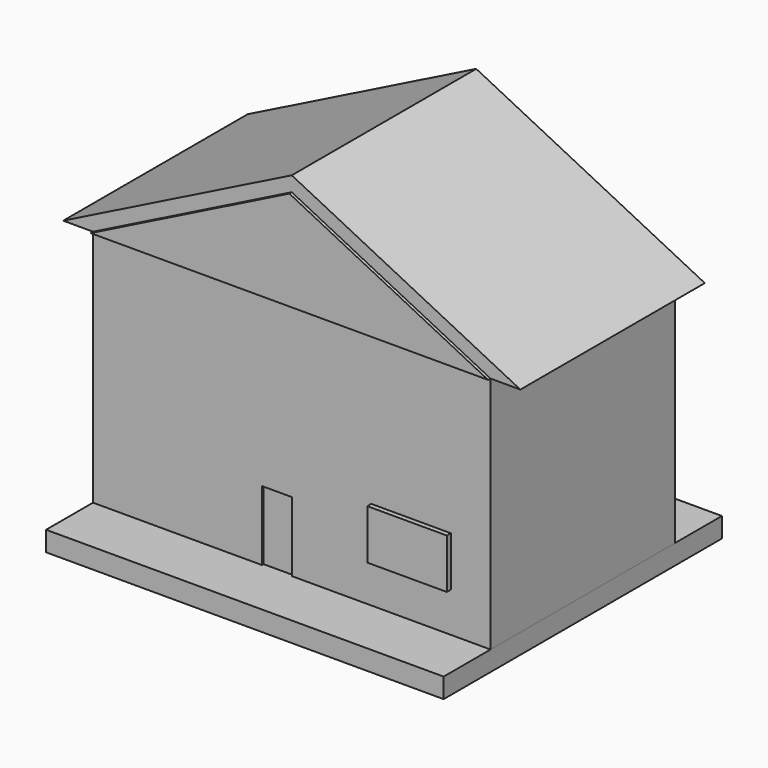
from build123d import *

# Parameters (mm, degrees)
F1_DEPTH     = 1066.8
F2_TEXT_SIZE = 1194.6976415647
F3_DEPTH     = 30.48
F4_DEPTH     = 3535.68
F5_DEPTH     = 3627.12
F0_W         = 2438.4
F0_H         = 1524
F6_DEPTH     = 3535.68
F7_DEPTH     = 5334
F0_W_2       = 914.4
F0_H_2       = 2133.6
F8_DEPTH     = 3474.72
F9_DEPTH     = 3688.08


# Not quite as in the source:
# - Text() gives the source's letters only with a copy of the font that has no kerning and outlines rounded to 1/6400 em; it was checked with that copy


with BuildPart() as f1:
    # F0 (on Front) → F1 (new body)
    with BuildSketch(Plane.XZ):
        Polygon((0, -609.6), (0, 0), (-6096, 0), (-7010.4, 0), (-12192, 0), (-12192, -609.6), align=None)
    extrude(amount=F1_DEPTH)

    # F2 (on face) → F3 (join)
    with BuildSketch(Plane.XY):
        with Locations((-11787.4422073364, -1066.8)):
            Text('Trevor Young', F2_TEXT_SIZE, font='Open Sans', text_align=(TextAlign.LEFT, TextAlign.BOTTOM))
    extrude(amount=F3_DEPTH)


with BuildPart() as f4:
    # F0 (on Front) → F4 (new body, symmetric)
    with BuildSketch(Plane.XZ):
        Polygon((-12192, 7315.2), (-6096, 10363.2), (-6096, 10820.4), (-13106.4, 7315.2), align=None)
        Polygon((-6096, 10363.2), (0, 7315.2), (914.4, 7315.2), (-6096, 10820.4), align=None)
    extrude(amount=F4_DEPTH, both=True)

    # F0 (on Front) → F5 (join, symmetric)
    with BuildSketch(Plane.XZ):
        Polygon((-12192, 7315.2), (-6096, 7315.2), (-6096, 10363.2), align=None)
        Polygon((-6096, 7315.2), (0, 7315.2), (-6096, 10363.2), align=None)
    extrude(amount=F5_DEPTH, both=True)


with BuildPart() as f6:
    # F0 (on Front) → F6 (new body, symmetric)
    with BuildSketch(Plane.XZ):
        Polygon((-6096, 0), (0, 0), (0, 7315.2), (-6096, 7315.2), (-12192, 7315.2), (-12192, 0), (-7010.4, 0), (-7010.4, 2133.6), (-6096, 2133.6), align=None)
        with Locations((-2438.4, 1981.2)):
            Rectangle(F0_W, F0_H, mode=Mode.SUBTRACT)
    extrude(amount=F6_DEPTH, both=True)

    # F0 (on Front) → F9 (join, symmetric)
    with BuildSketch(Plane.XZ):
        with Locations((-2438.4, 1981.2)):
            Rectangle(F0_W, F0_H)
    extrude(amount=F9_DEPTH, both=True)


with BuildPart() as f7:
    # F0 (on Front) → F7 (new body, symmetric)
    with BuildSketch(Plane.XZ):
        Polygon((0, -609.6), (0, 0), (-6096, 0), (-7010.4, 0), (-12192, 0), (-12192, -609.6), align=None)
    extrude(amount=F7_DEPTH, both=True)


with BuildPart() as f8:
    # F0 (on Front) → F8 (new body, symmetric)
    with BuildSketch(Plane.XZ):
        with Locations((-6553.2, 1066.8)):
            Rectangle(F0_W_2, F0_H_2)
    extrude(amount=F8_DEPTH, both=True)


solid = Compound([f1.part, f4.part, f6.part, f7.part, f8.part])
